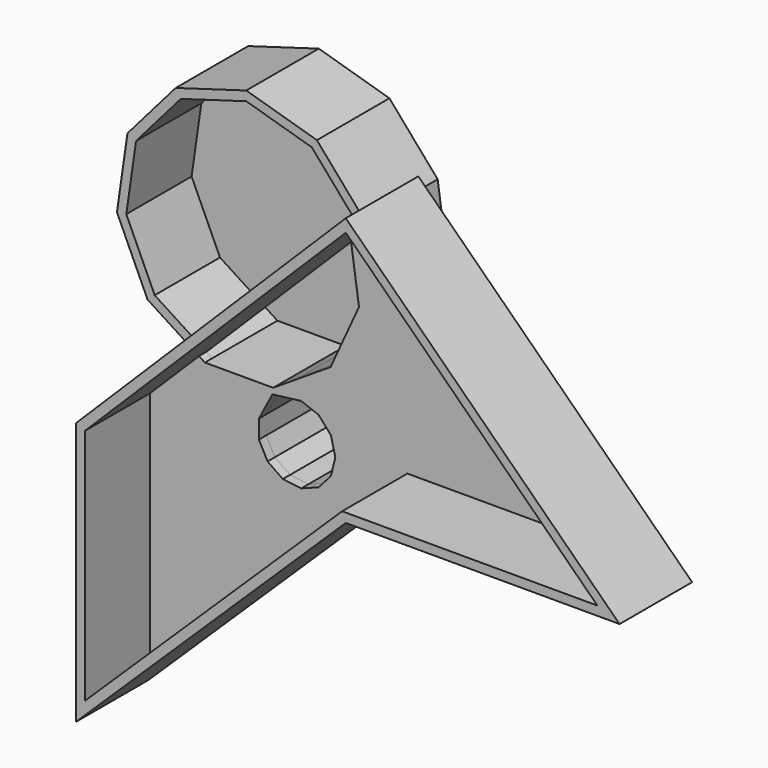
from build123d import *

# Parameters (mm, degrees)
F1_DEPTH     = 25.4
F2_T         = -2.54
F4_DEPTH     = 25.4
F5_T         = 2.54
F5_T3_DEPTH  = 30.48
F5_T5_DEPTH  = 10.9375095944
F5_T7_DEPTH  = 21.4331791904
F5_T9_DEPTH  = 11.5273250997
F5_T11_DEPTH = 11.5273250997
F5_T13_DEPTH = 11.5273250997
F5_T15_DEPTH = 11.5273250997
F5_T17_DEPTH = 11.5273250997
F5_T19_DEPTH = 11.5273250997
F5_T21_DEPTH = 11.5273250997
F5_T23_DEPTH = 11.5273250997
F5_T25_DEPTH = 11.5273250997
F5_T27_DEPTH = 11.5273250997
F5_T29_DEPTH = 11.5273250997
F5_T31_DEPTH = 5.7399744024
F5_T33_DEPTH = 17.6352883916
F5_T35_DEPTH = 25.6999516571
F5_T37_DEPTH = 25.6999516571
F5_T39_DEPTH = 5.8481406641
F5_T41_DEPTH = 30.48
F5_T43_DEPTH = 27.94


# Not quite as in the source:
# - a shell that OpenCascade refuses in one call is made with other operations: the cavity is built on its own and cut out


with BuildPart() as f1:
    # F0 (on Front) → F1 (new body)
    with BuildSketch(Plane.XZ):
        Polygon((76.6998529434, 0), (0, 75.1383975148), (-75.6014883518, 0), (-75.6014883518, -73.6595392227), (0, 0), align=None)
    extrude(amount=F1_DEPTH)

    # F2
    f2_openings = [f1.faces().sort_by_distance(p)[0] for p in [
        (-16.251734, -25.4, 8.81054),
    ]]
    offset(amount=F2_T, openings=f2_openings, kind=Kind.INTERSECTION)

    # F3 (on face) → F4 (join)
    with BuildSketch(Plane(origin=(0, 0, 0), x_dir=(-1, 0, 0), z_dir=(0, 1, 0))):
        Polygon((45.1430156827, -3.2236625498), (45.1430156827, 3.2236625498), (42.1467943112, 8.9324854087), (37.8800218445, 8.9324854087), (31.0955953813, 13.2925715491), (30.4404329353, 13.3721226726), (24.4120792452, 11.0858696839), (20.1367118865, 6.2599775498), (18.5937659974, 0), (20.1367118865, -6.2599775498), (24.4120792452, -11.0858696839), (30.4404329353, -13.3721226726), (36.8407497759, -12.5949835086), (42.1467943112, -8.9324854087), align=None)
        Polygon((37.8800218445, 8.9324854087), (42.1467943112, 8.9324854087), (36.8407497759, 12.5949835086), (31.0955953813, 13.2925715491), align=None)
        Polygon((36.8407497759, 12.5949835086), (42.1467943112, 8.9324854087), (58.4999735016, 8.9324854087), (75.8465806799, 20.0804729285), (84.4124181657, 38.8370406985), (81.4778930804, 59.2471109792), (67.9746964043, 74.8306306673), (48.189997673, 80.6399423696), (28.4052989418, 74.8306306673), (14.9021022657, 59.2471109792), (11.9675771804, 38.8370406985), (20.5334146661, 20.0804729285), (31.0955953813, 13.2925715491), align=None)
    extrude(amount=F4_DEPTH)

    # F5: shell of thickness 2.54, made by hand


with BuildPart() as f5_core1:
    # F5_t2: copy of F1
    add(f1.part)

    # the walls: a layer under each face that stays
    f5_faces = [f5_core1.faces().sort_by_distance(p)[0] for p in [
        (38.3499264717, -12.7, 37.5691987574),
        (38.3499264717, -12.7, 0),
        (-37.8007441759, -12.7, 37.5691987574),
        (0.5491822958, 0, 0.7394291461),
        (0.5491822958, -25.4, 0.7394291461),
        (-37.8007441759, -12.7, -36.8297696114),
        (-75.6014883518, -12.7, -36.8297696114),
        (-67.1732770908, 12.7, 14.5064791686),
        (-50.3233839064, 12.7, 8.9324854087),
        (-43.6449049969, 12.7, 6.0780739793),
        (-45.1430156827, 12.7, 0),
        (-43.6449049969, 12.7, -6.0780739793),
        (-39.4937720436, 12.7, -10.7637344586),
        (-33.6405913556, 12.7, -12.9835530906),
        (-27.4262560902, 12.7, -12.2289961783),
        (-22.2743955659, 12.7, -8.6729236169),
        (-19.365238942, 12.7, -3.1299887749),
        (-19.365238942, 12.7, 3.1299887749),
        (-22.2743955659, 12.7, 8.6729236169),
        (-27.4262560902, 12.7, 12.2289961783),
        (-30.7680141583, 12.7, 13.3323471109),
        (-25.8145050237, 12.7, 16.6865222388),
        (-16.2504959233, 12.7, 29.4587568135),
        (-13.434839723, 12.7, 49.0420758389),
        (-21.6537006037, 12.7, 67.0388708233),
        (35.245158445, -13.97, 37.0550334809),
        (34.7223268727, -13.97, 2.54),
        (-37.0471427298, -13.97, -32.5492576556),
        (-73.0614883518, -13.97, -34.3475958286),
        (-36.5243111575, -13.97, 35.2566953079),
        (-38.2976483074, 12.7, 77.7352865185),
        (-58.0823470387, 12.7, 77.7352865185),
        (-74.7262947424, 12.7, 67.0388708233),
        (-82.945155623, 12.7, 49.0420758389),
        (-80.1294994228, 12.7, 29.4587568135),
        (-48.189997673, 25.4, 33.6339098485),
    ]]
    thicken(f5_faces, amount=-F5_T, mode=Mode.SUBTRACT)

    # F5_s4 → F5_t3 (cut)
    with BuildSketch(Plane.XZ.offset(-2.54)):
        Polygon((0.0177253382, -0.0435926464), (0, 2.54), (-1.0327971077, 2.54), (-1.7725338247, 1.8192646427), align=None)
    extrude(amount=F5_T3_DEPTH, mode=Mode.SUBTRACT)

    # F5_s6 → F5_t5 (cut)
    with BuildSketch(Plane(origin=(-43.3267236667, 0, 27.8443945691), x_dir=(0, 1, 0), z_dir=(-0.8412535328, 0, 0.5406408175))):
        Polygon((0.0254, 24.138388588), (-2.54, 24.112988588), (-2.54, 21.572988588), (0, 21.572988588), align=None)
    extrude(amount=F5_T5_DEPTH, mode=Mode.SUBTRACT)

    # F5_s8 → F5_t7 (cut)
    with BuildSketch(Plane.YZ.offset(-61.0399735016)):
        Polygon((0.0254, 8.9070854087), (-2.54, 8.9324854087), (-2.54, 11.4724854087), (0, 11.4724854087), align=None)
    extrude(amount=F5_T7_DEPTH, mode=Mode.SUBTRACT)

    # F5_s10 → F5_t9 (cut)
    with BuildSketch(Plane(origin=(-9.6033156793, 0, -18.2975892876), x_dir=(0, 1, 0), z_dir=(0.464723172, 0, 0.8854560257))):
        Polygon((0.0254, 41.4956659382), (-2.54, 41.4702659382), (-2.54, 38.9302659382), (0, 38.9302659382), align=None)
    extrude(amount=F5_T9_DEPTH, mode=Mode.SUBTRACT)

    # F5_s12 → F5_t11 (cut)
    with BuildSketch(Plane.XY.offset(-5.7636625498)):
        Polygon((-45.1684156827, 0.0254), (-45.1430156827, -2.54), (-42.6030156827, -2.54), (-42.6030156827, 0), align=None)
    extrude(amount=F5_T11_DEPTH, mode=Mode.SUBTRACT)

    # F5_s14 → F5_t13 (cut)
    with BuildSketch(Plane(origin=(-4.2463005938, 0, 8.0906498184), x_dir=(0, 1, 0), z_dir=(-0.464723172, 0, 0.8854560257))):
        Polygon((0.0254, 41.4956659382), (-2.54, 41.4702659382), (-2.54, 38.9302659382), (0, 38.9302659382), align=None)
    extrude(amount=F5_T13_DEPTH, mode=Mode.SUBTRACT)

    # F5_s16 → F5_t15 (cut)
    with BuildSketch(Plane(origin=(-16.9736937466, 0, 11.7160948578), x_dir=(0, 1, 0), z_dir=(-0.8229838659, 0, 0.5680647467))):
        Polygon((0.0254, 31.3187994096), (-2.54, 31.2933994096), (-2.54, 28.7533994096), (0, 28.7533994096), align=None)
    extrude(amount=F5_T15_DEPTH, mode=Mode.SUBTRACT)

    # F5_s18 → F5_t17 (cut)
    with BuildSketch(Plane(origin=(-25.876601356, 0, 3.1419882557), x_dir=(0, 1, 0), z_dir=(-0.9927088741, 0, 0.1205366803))):
        Polygon((0.0254, 16.9692135742), (-2.54, 16.9438135742), (-2.54, 14.4038135742), (0, 14.4038135742), align=None)
    extrude(amount=F5_T17_DEPTH, mode=Mode.SUBTRACT)

    # F5_s20 → F5_t19 (cut)
    with BuildSketch(Plane(origin=(-22.6430959031, 0, -8.5873935644), x_dir=(0, 1, 0), z_dir=(-0.9350162427, 0, -0.354604887))):
        Polygon((0.0254, 1.7342256155), (-2.54, 1.7088256155), (-2.54, -0.8311743845), (0, -0.8311743845), align=None)
    extrude(amount=F5_T19_DEPTH, mode=Mode.SUBTRACT)

    # F5_s22 → F5_t21 (cut)
    with BuildSketch(Plane(origin=(-10.277585823, 0, -11.6009962232), x_dir=(0, 1, 0), z_dir=(-0.6631226582, 0, -0.7485107482))):
        Polygon((0.0254, -10.8960123265), (-2.54, -10.9214123265), (-2.54, -13.4614123265), (0, -13.4614123265), align=None)
    extrude(amount=F5_T21_DEPTH, mode=Mode.SUBTRACT)

    # F5_s24 → F5_t23 (cut)
    with BuildSketch(Plane(origin=(-0.4570401404, 0, -1.854284741), x_dir=(0, 1, 0), z_dir=(-0.2393156643, 0, -0.9709418174))):
        Polygon((0.0254, -18.0280649503), (-2.54, -18.0534649503), (-2.54, -20.5934649503), (0, -20.5934649503), align=None)
    extrude(amount=F5_T23_DEPTH, mode=Mode.SUBTRACT)

    # F5_s26 → F5_t25 (cut)
    with BuildSketch(Plane(origin=(-3.2157096041, 0, 13.0466467234), x_dir=(0, 1, 0), z_dir=(0.2393156643, 0, -0.9709418174))):
        Polygon((0.0254, -18.0280649503), (-2.54, -18.0534649503), (-2.54, -20.5934649503), (0, -20.5934649503), align=None)
    extrude(amount=F5_T25_DEPTH, mode=Mode.SUBTRACT)

    # F5_s28 → F5_t27 (cut)
    with BuildSketch(Plane(origin=(-17.9216162855, 0, 20.229322958), x_dir=(0, 1, 0), z_dir=(0.6631226582, 0, -0.7485107482))):
        Polygon((0.0254, -10.8960123265), (-2.54, -10.9214123265), (-2.54, -13.4614123265), (0, -13.4614123265), align=None)
    extrude(amount=F5_T27_DEPTH, mode=Mode.SUBTRACT)

    # F5_s30 → F5_t29 (cut)
    with BuildSketch(Plane(origin=(-33.4213321061, 0, 12.6750393793), x_dir=(0, 1, 0), z_dir=(0.9350162427, 0, -0.354604887))):
        Polygon((0.0254, 1.7342256155), (-2.54, 1.7088256155), (-2.54, -0.8311743845), (0, -0.8311743845), align=None)
    extrude(amount=F5_T29_DEPTH, mode=Mode.SUBTRACT)

    # F5_s32 → F5_t31 (cut)
    with BuildSketch(Plane(origin=(-31.5747248824, 0, -3.8338657149), x_dir=(0, 1, 0), z_dir=(0.9927088741, 0, 0.1205366803))):
        Polygon((0.0254, 16.9692135742), (-2.54, 16.9438135742), (-2.54, 14.4038135742), (0, 14.4038135742), align=None)
    extrude(amount=F5_T31_DEPTH, mode=Mode.SUBTRACT)

    # F5_s34 → F5_t33 (cut)
    with BuildSketch(Plane(origin=(-3.2619473911, 0, -2.0963262978), x_dir=(0, 1, 0), z_dir=(-0.8412535328, 0, -0.5406408175))):
        Polygon((0.0254, -27.9685708823), (-2.54, -27.9939708823), (-2.54, -30.5339708823), (0, -30.5339708823), align=None)
    extrude(amount=F5_T33_DEPTH, mode=Mode.SUBTRACT)

    # F5_s36 → F5_t35 (cut)
    with BuildSketch(Plane(origin=(13.6654522193, 0, 29.9231664254), x_dir=(0, 1, 0), z_dir=(-0.415415013, 0, -0.9096319954))):
        Polygon((0.0254, -26.9941808769), (-2.54, -27.0195808769), (-2.54, -29.5595808769), (0, -29.5595808769), align=None)
    extrude(amount=F5_T35_DEPTH, mode=Mode.SUBTRACT)

    # F5_s38 → F5_t37 (cut)
    with BuildSketch(Plane(origin=(-9.0092196449, 0, 62.6604989846), x_dir=(0, 1, 0), z_dir=(0.1423148383, 0, -0.9898214419))):
        Polygon((0.0254, -6.2932773345), (-2.54, -6.3186773345), (-2.54, -8.8586773345), (0, -8.8586773345), align=None)
    extrude(amount=F5_T37_DEPTH, mode=Mode.SUBTRACT)

    # F5_s40 → F5_t39 (cut)
    with BuildSketch(Plane(origin=(-37.8790578276, 0, 43.7147630729), x_dir=(0, 1, 0), z_dir=(0.6548607339, 0, -0.7557495744))):
        Polygon((0.0254, 27.5617491357), (-2.54, 27.5363491357), (-2.54, 24.9963491357), (0, 24.9963491357), align=None)
    extrude(amount=F5_T39_DEPTH, mode=Mode.SUBTRACT)

    # F5_s42 → F5_t41 (cut)
    with BuildSketch(Plane.XZ.offset(-27.94)):
        Polygon((-42.1692848942, 8.9188893773), (-42.1467943112, 11.4724854087), (-37.9451211064, 11.4724854087), (-39.897736006, 7.7520885517), align=None)
        Polygon((-31.0849247362, 13.2964185148), (-30.7894322134, 10.7710910089), (-41.7969422831, 9.4345373059), (-32.4688230576, 15.4293555225), align=None)
    extrude(amount=F5_T41_DEPTH, mode=Mode.SUBTRACT)

    # F5_s44 → F5_t43 (cut)
    with BuildSketch(Plane.XZ):
        Polygon((70.4596759808, 2.5472557471), (72.254938082, 4.3544252949), (76.6998529434, 0), (70.4774508531, 0), align=None)
        Polygon((0.0129964155, 71.5339071047), (1.7903532658, 73.3844922566), (0, 75.1383975148), (-1.7776590552, 73.3716273672), align=None)
        Polygon((-73.0538136901, -67.6203226649), (-71.2889545271, -69.457779954), (-75.6014883518, -73.6595392227), (-75.6014883518, -67.6385153113), align=None)
        Polygon((-73.0181831009, -1.0746919499), (-75.6014883518, -1.0566763458), (-75.6014883518, 0), (-74.8520134439, 0.7448840596), align=None)
    extrude(amount=F5_T43_DEPTH, mode=Mode.SUBTRACT)


with BuildPart() as f1_1:
    add(f1.part)

    # what is left inside the walls is the cavity
    f5_cavity = [f5_core1.part.solids().sort_by_distance(p)[0] for p in [
        (-48.189998, 22.8346, 33.645894),
        (-31.906399, 22.8346, -3.591727),
    ]]
    add(f5_cavity, mode=Mode.SUBTRACT)


solid = f1_1.part
